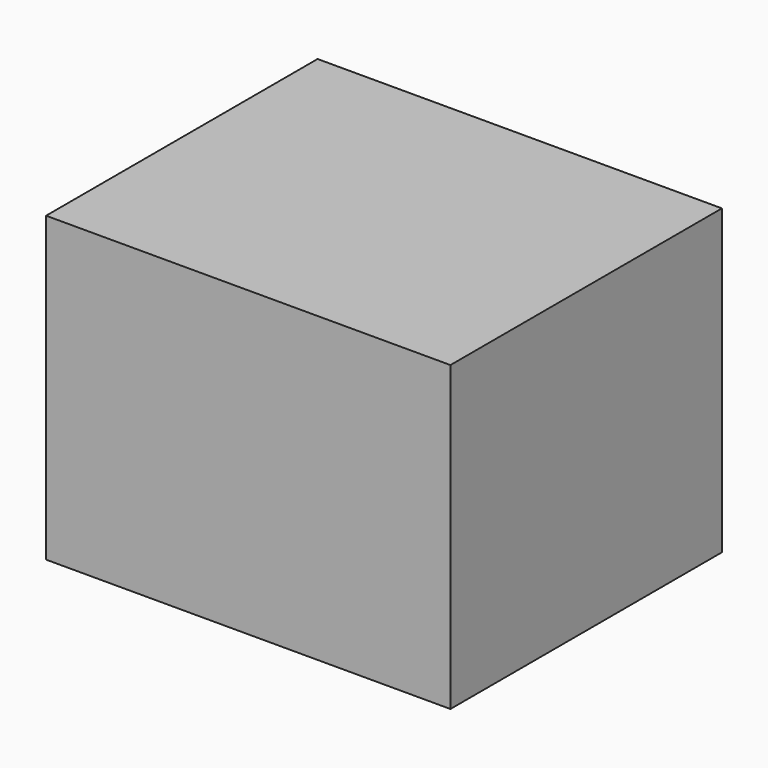
from build123d import *

# Parameters (mm, degrees)
F1_W     = 69.7055906057
F1_H     = 58.5029125214
F2_DEPTH = 52.1997734904


# Not quite as in the source:
# - the program builds the solid bodies; features that only make, move or delete a surface that nothing else refers to are left out


with BuildPart() as f2:
    # F1 (on face) → F2 (new body)
    with BuildSketch(Plane.XY):
        with Locations((2.4894550443, 1.037299633)):
            Rectangle(F1_W, F1_H)
    extrude(amount=F2_DEPTH)


solid = f2.part
